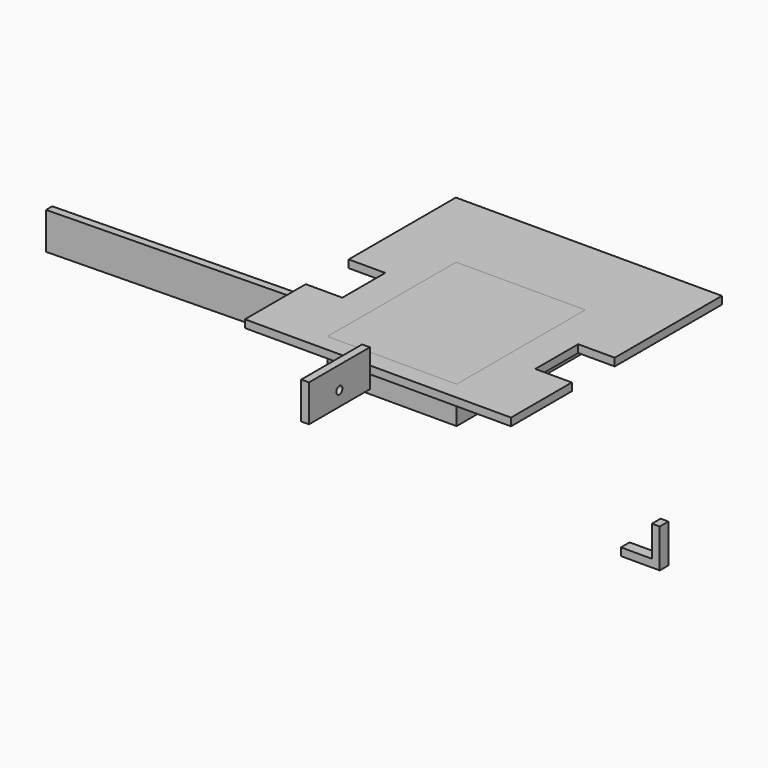
from build123d import *

# Parameters (mm, degrees)
F0_W          = 53
F0_H          = 66
F3_DEPTH      = 3.175
F1_W          = 31.2166
F1_H          = 15.1638
F1_R          = 1.5875
F4_DEPTH      = 3.175
F1_W_2        = 54.9460835755
F5_DEPTH      = 3.175
F6_DEPTH      = 3.175
F7_DEPTH      = 3.175
F7_DEPTH_BACK = 12
F8_DEPTH      = 4.445


# Not quite as in the source:
# - a length typed as a fraction of an inch, garbled in the dataset ("3 / 203.2 mm" for 3/8 in), is restored


with BuildPart() as f3:
    # F0 (on Top) → F3 (new body)
    with BuildSketch(Plane.XY):
        Polygon((-54.5999980115, -22), (-54.5999980115, -53.2168401558), (54.5999980115, -53.2168401558), (54.5999980115, -21.9964), (39.5999980115, -21.9964), (39.5999980115, 0), (54.5999980115, 0), (54.5999980115, 54.9831558671), (-54.5999980115, 54.9831558671), (-54.5999980115, 0), (-39.5999980115, 0), (-39.5999980115, -22), align=None)
        with Locations((0, -13)):
            Rectangle(F0_W, F0_H, mode=Mode.SUBTRACT)
    extrude(amount=F3_DEPTH)


with BuildPart() as f4:
    # F1 (on Right) → F4 (new body)
    with BuildSketch(Plane.YZ):
        with Locations((-76.9739231968, 7.5819)):
            Rectangle(F1_W, F1_H)
        with Locations((-76.9739231968, 6)):
            Circle(F1_R, mode=Mode.SUBTRACT)
    extrude(amount=F4_DEPTH)


with BuildPart() as f5:
    # F1 (on Right) → F5 (new body)
    with BuildSketch(Plane.YZ):
        with Locations((43.6124540865, -22.5870617241)):
            Rectangle(F1_W_2, F1_H)
    extrude(amount=F5_DEPTH)


with BuildPart() as f6:
    # F2 (on Front) → F6 (new body)
    with BuildSketch(Plane.XZ):
        Polygon((-60.7066550265, -15.606769852), (-176.2403489556, -17.194269852), (-176.2403489556, -32.358069852), (-60.7066550265, -30.770569852), align=None)
    extrude(amount=F6_DEPTH)


with BuildPart() as f7:
    # F0 (on Top) → F7 (new body, two sides)
    with BuildSketch(Plane.XY) as f7_sk:
        with Locations((0, -13)):
            Rectangle(F0_W, F0_H)
    extrude(amount=F7_DEPTH)
    extrude(f7_sk.sketch, amount=-F7_DEPTH_BACK)


with BuildPart() as f8:
    # F2 (on Front) → F8 (new body)
    with BuildSketch(Plane.XZ):
        Polygon((76.5899116695, -48.8504437208), (73.4149116695, -48.8504437208), (73.4149116695, -61.5504437208), (60.7149116695, -61.5504437208), (60.7149116695, -64.7254437208), (76.6233354807, -64.7254437208), align=None)
    extrude(amount=F8_DEPTH)


solid = Compound([f3.part, f4.part, f5.part, f6.part, f7.part, f8.part])
